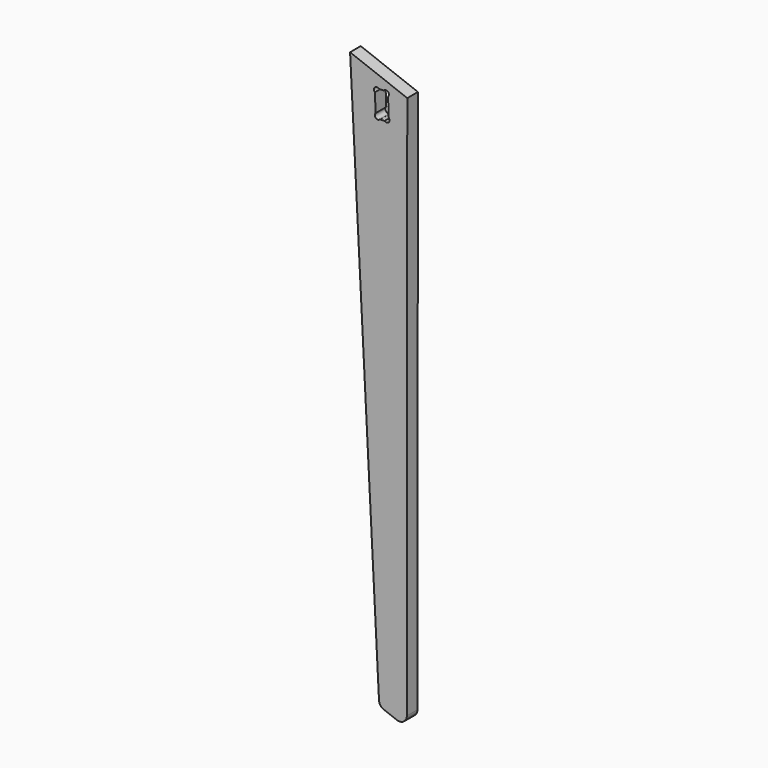
from build123d import *

# Parameters (mm, degrees)
F0_R     = 3
F1_DEPTH = 18
F2_DEPTH = 14


# Not quite as in the source:
# - ends of sketch curves that miss each other by under 0.0002 mm in the source are joined


with BuildPart() as f1:
    # F0 (on Front) → F1 (new body)
    with BuildSketch(Plane.XZ):
        with BuildLine():
            Line((-42.3895305789, -243.8882939158), (-24.7354158314, -250.6203213983))
            ThreePointArc((-24.7354158314, -250.6203213983), (-15.5028330705, -249.5140993631), (-11.1723924415, -241.2853938543))
            Line((-11.1723924415, -241.2853938543), (-10.5257942379, 495.2740080398))
            Line((-10.5257942379, 495.2740080398), (-87.9671722006, 524.8046568947))
            Line((-87.9671722006, 524.8046568947), (-48.8132548023, -235.0591811233))
            ThreePointArc((-48.8132548023, -235.0591811233), (-46.9127527413, -240.4278329279), (-42.3895305789, -243.8882939158))
        make_face()
        with Locations((-27.881012126, -192.8539189117)):
            Circle(F0_R, mode=Mode.SUBTRACT)
        with Locations((-30.5399937075, -49.059701124)):
            Circle(F0_R, mode=Mode.SUBTRACT)
        with Locations((-35.8245981399, 119.2769033151)):
            Circle(F0_R, mode=Mode.SUBTRACT)
        with Locations((-37.6148353963, 326.2889456799)):
            Circle(F0_R, mode=Mode.SUBTRACT)
        with BuildLine():
            ThreePointArc((-35.8713849562, 463.9863896495), (-35.6237850386, 458.3139596858), (-41.2978981422, 458.1085140717))
            Line((-41.2978981422, 458.1085140717), (-47.5773687005, 457.9045057833))
            ThreePointArc((-47.5773687005, 457.9045057833), (-53.2508540354, 457.7393262229), (-53.3777836629, 463.4137960782))
            Line((-53.3777836629, 463.4137960782), (-54.3935717097, 487.9983330149))
            ThreePointArc((-54.3935717097, 487.9983330149), (-54.636241933, 493.6693642066), (-48.9636796908, 493.8731318846))
            Line((-48.9636796908, 493.8731318846), (-42.2828997396, 494.0973559272))
            ThreePointArc((-42.2828997396, 494.0973559272), (-36.6071005964, 494.2603360531), (-36.4869165759, 488.5834695431))
            Line((-36.4869165759, 488.5834695431), (-35.8713849562, 463.9863896495))
        make_face(mode=Mode.SUBTRACT)
        with Locations((-43.7681841537, 431.407725542)):
            Circle(F0_R, mode=Mode.SUBTRACT)
        with Locations((-23.2091454593, 473.1308742023)):
            Circle(F0_R, mode=Mode.SUBTRACT)
        with Locations((-43.7681841537, 431.407725542)):
            Circle(F0_R)
        with Locations((-23.2091454593, 473.1308742023)):
            Circle(F0_R)
        with Locations((-37.6148353963, 326.2889456799)):
            Circle(F0_R)
        with Locations((-35.8245981399, 119.2769033151)):
            Circle(F0_R)
        with Locations((-27.881012126, -192.8539189117)):
            Circle(F0_R)
        with Locations((-30.5399937075, -49.059701124)):
            Circle(F0_R)
    extrude(amount=F1_DEPTH)

    # F0 (on Front) → F2 (cut)
    with BuildSketch(Plane.XZ):
        with Locations((-43.7681841537, 431.407725542)):
            Circle(F0_R)
        with Locations((-23.2091454593, 473.1308742023)):
            Circle(F0_R)
        with Locations((-37.6148353963, 326.2889456799)):
            Circle(F0_R)
        with Locations((-35.8245981399, 119.2769033151)):
            Circle(F0_R)
        with Locations((-27.881012126, -192.8539189117)):
            Circle(F0_R)
        with Locations((-30.5399937075, -49.059701124)):
            Circle(F0_R)
    extrude(amount=F2_DEPTH, mode=Mode.SUBTRACT)


solid = f1.part
